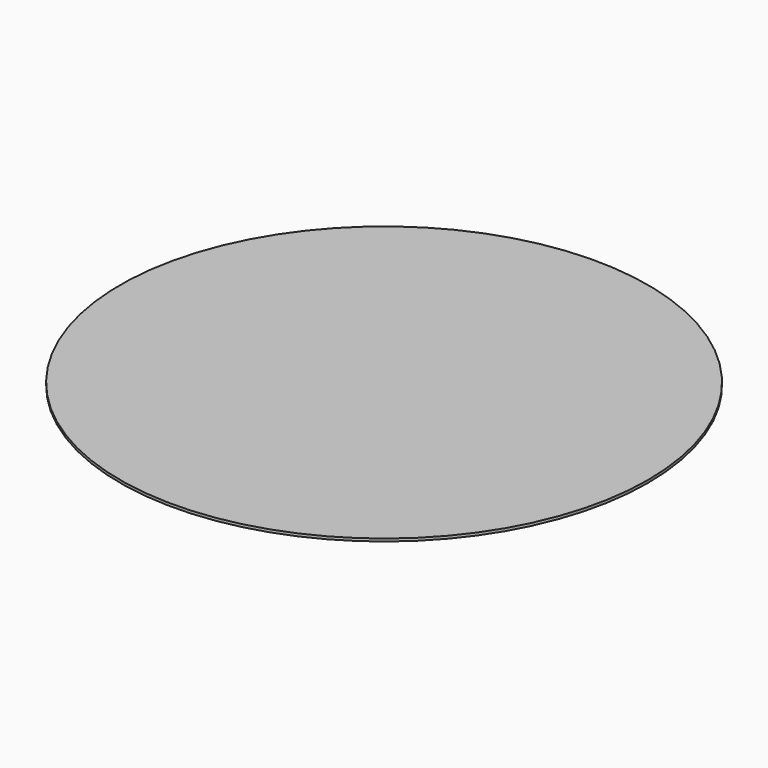
from build123d import *

# Parameters (mm, degrees)
F0_R     = 200
F2_DEPTH = 102
F3_DEPTH = 100


# Not quite as in the source:
# - the program builds the solid bodies; features that only make, move or delete a surface that nothing else refers to are left out


with BuildPart() as f2:
    # F0 (on Top) → F2 (new body)
    with BuildSketch(Plane.XY):
        Circle(F0_R)
    extrude(amount=-F2_DEPTH)

    # F0 (on Top) → F3 (cut)
    with BuildSketch(Plane.XY):
        Circle(F0_R)
    extrude(amount=-F3_DEPTH, mode=Mode.SUBTRACT)


solid = f2.part
